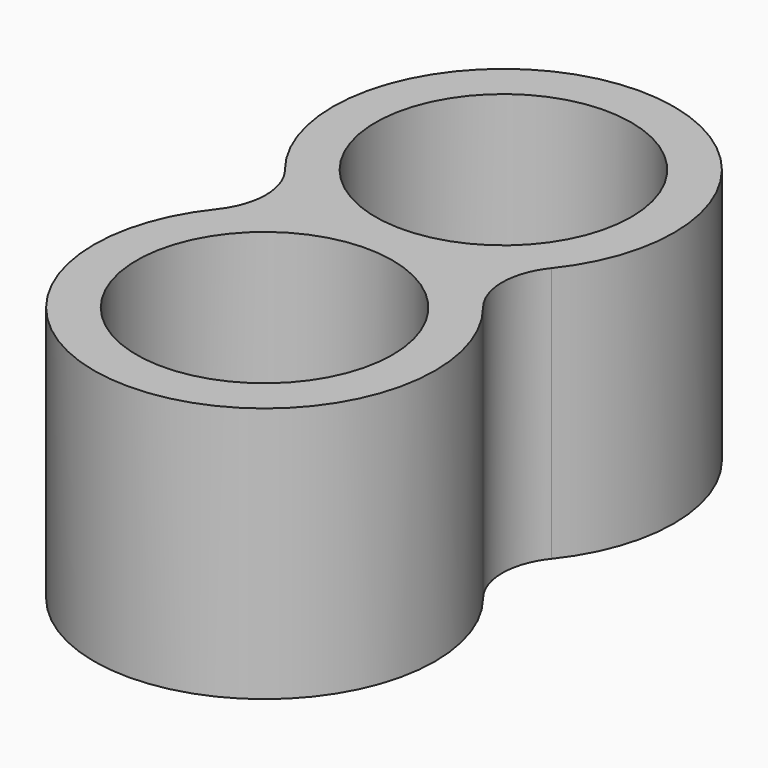
from build123d import *

# Parameters (mm, degrees)
F0_R     = 9.525
F1_DEPTH = 19.05
F2_R     = 5.08


with BuildPart() as f1:
    # F0 (on Top) → F1 (new body)
    with BuildSketch(Plane.XY):
        with BuildLine():
            ThreePointArc((-6.1483610621, -11.1125), (0, -34.925), (6.1483610621, -11.1125))
            ThreePointArc((6.1483610621, -11.1125), (0, 12.7), (-6.1483610621, -11.1125))
        make_face()
        with Locations((0, -22.225)):
            Circle(F0_R, mode=Mode.SUBTRACT)
        Circle(F0_R, mode=Mode.SUBTRACT)
    extrude(amount=F1_DEPTH)

    # F2
    f2_edges = [f1.edges().sort_by_distance(p)[0] for p in [
        (6.148361, -11.1125, 9.525),
        (-6.148361, -11.1125, 9.525),
    ]]
    fillet(f2_edges, radius=F2_R)


solid = f1.part
